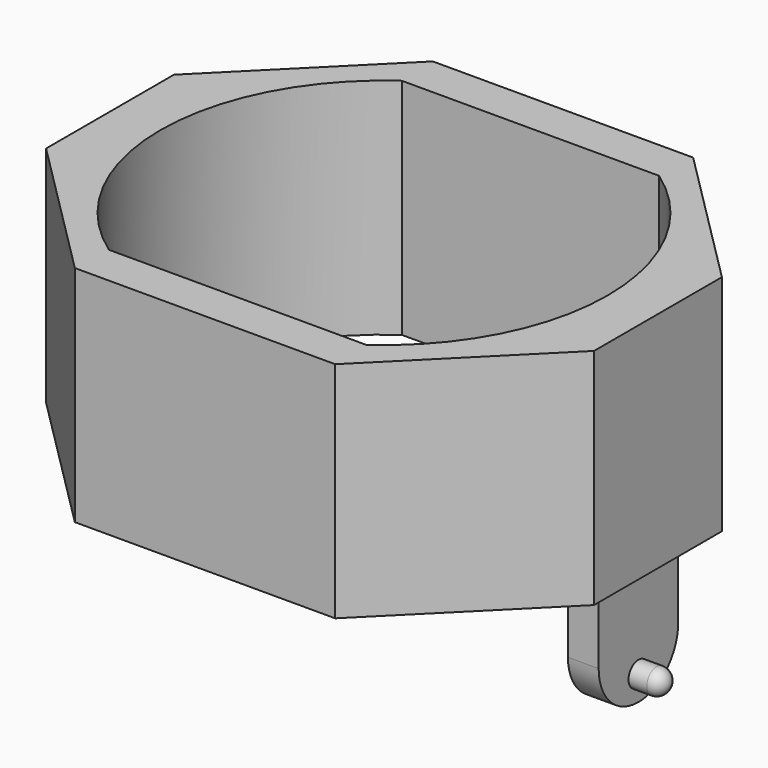
from build123d import *

# Parameters (mm, degrees)
F1_DEPTH  = 22.86
F3_DEPTH  = 6.35
F4_R      = 0.635
F5_DEPTH  = 1.5691231
F6_R      = 2.53999
F7_R      = 0.635
F9_DEPTH  = 6.35
F11_D     = 2.54
F16_D     = 127
F16_DEPTH = 17.781


# Not quite as in the source:
# - a fillet or chamfer is up to 0.001 mm smaller than in the source, because OpenCascade refuses the exact size
# - a length typed as a fraction of an inch, garbled in the dataset ("3 / 203.2 mm" for 3/8 in), is restored
# - the program builds the solid bodies; features that only make, move or delete a surface that nothing else refers to are left out


with BuildPart() as f1:
    # F0 (on Top) → F1 (new body)
    with BuildSketch(Plane.XY):
        Polygon((6.6501818182, 11.43), (0, 11.43), (-6.6501818182, 11.43), (-13.9976640991, 4.0825177191), (-13.9976640991, 0), (-13.9976640991, -4.0825177191), (-6.6501818182, -11.43), (0, -11.43), (6.6501818182, -11.43), (13.9976640991, -4.0825177191), (13.9976640991, 0), (13.9976640991, 4.0825177191), align=None)
        with BuildLine():
            ThreePointArc((6.5717879374, 9.3518181818), (10.1429886159, 5.26922024), (11.43, 0))
            ThreePointArc((11.43, 0), (10.1429886159, -5.26922024), (6.5717879374, -9.3518181818))
            Line((6.5717879374, -9.3518181818), (0, -9.3518181818))
            Line((0, -9.3518181818), (-6.5717879374, -9.3518181818))
            ThreePointArc((-6.5717879374, -9.3518181818), (-10.1429886159, -5.26922024), (-11.43, 0))
            ThreePointArc((-11.43, 0), (-10.1429886159, 5.26922024), (-6.5717879374, 9.3518181818))
            Line((-6.5717879374, 9.3518181818), (0, 9.3518181818))
            Line((0, 9.3518181818), (6.5717879374, 9.3518181818))
        make_face(mode=Mode.SUBTRACT)
    extrude(amount=F1_DEPTH)

    # F2 (on Top) → F3 (join)
    with BuildSketch(Plane.XY):
        Polygon((12.9991231, -2.54), (12.9991231, 0), (12.9991231, 2.54), (11.43, 2.54), (11.43, 0), (11.43, -2.54), align=None)
    extrude(amount=-F3_DEPTH)

    # F4 (on face) → F5 (join)
    with BuildSketch(Plane.YZ.offset(12.9991231)):
        with Locations((0, -5.08)):
            Circle(F4_R)
    extrude(amount=F5_DEPTH)

    # F6 (radius 2.54 in the source; OpenCascade refuses exactly that, so slightly less here)
    f6_edges = [f1.edges().sort_by_distance(p)[0] for p in [
        (12.214562, -2.54, -6.35),
        (12.214562, 2.54, -6.35),
    ]]
    fillet(f6_edges, radius=F6_R)

    # F7
    f7_edges = [f1.edges().sort_by_distance(p)[0] for p in [
        (14.568246, -0.635, -5.08),
    ]]
    fillet(f7_edges, radius=F7_R)

    # F8 (on face) → F9 (join)
    with BuildSketch(Plane.XY.offset(22.86)):
        Polygon((13.9976640991, 2.54), (12.4285360385, 2.54), (12.4285360385, 0), (12.4285360385, -2.54), (13.9976640991, -2.54), (13.9976640991, 0), align=None)
    extrude(amount=F9_DEPTH)

    # F11 (through all)
    with Locations(Plane.YZ.offset(13.9976640991)):
        with Locations((0, 26.67)):
            Hole(F11_D / 2)

    # F12: F1 across plane


with BuildPart() as f1_1:
    add(f1.part)
    add(f1.part.mirror(Plane.YZ))

    # F16 (through all, one way)
    with BuildSketch(Plane(origin=(0, 0, 11.43), x_dir=(1, 0, 0), z_dir=(0, 0, -1))):
        with Locations((0, 0)):
            Circle(F16_D / 2)
    extrude(amount=-F16_DEPTH, mode=Mode.SUBTRACT)


solid = f1_1.part
